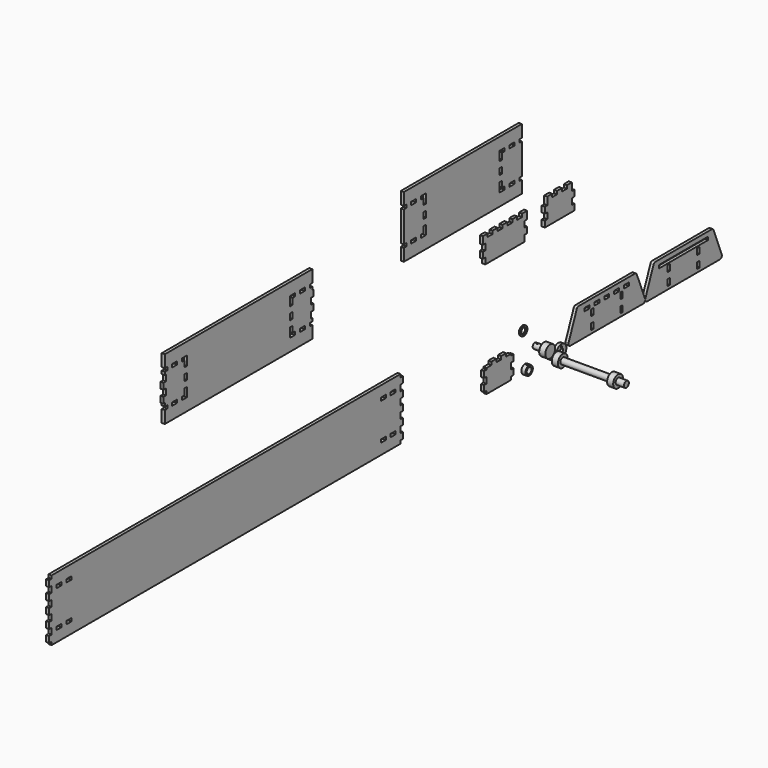
from build123d import *

# Parameters (mm, degrees)
F0_W      = 152.4
F0_H      = 101.6
F0_W_2    = 6.35
F0_H_2    = 12.7
F1_DEPTH  = 6.35
F2_W      = 152.4
F2_H      = 101.6
F2_W_2    = 6.35
F2_H_2    = 12.7
F2_W_3    = 127
F2_H_3    = 6.35
F3_DEPTH  = 6.35
F5_DEPTH  = 6.35
F6_W      = 12.7
F6_H      = 6.35
F7_DEPTH  = 6.35
F8_R      = 5.715
F9_DEPTH  = 19.05
F10_R     = 5.715
F11_DEPTH = 17.145
F12_R     = 12.7
F12_R_2   = 5.715
F13_DEPTH = 12.7
F14_R     = 6.35
F15_DEPTH = 101.6
F16_R     = 12.7
F16_R_2   = 6.35
F17_DEPTH = 12.7
F18_R     = 6.35
F19_DEPTH = 17.145
F20_R     = 12.7
F20_R_2   = 5.715
F21_DEPTH = 12.7
F22_R     = 1.5875
F23_DEPTH = 127.001
F24_R     = 9.525
F25_DEPTH = 8.4666666667
F26_R     = 1.5875
F27_DEPTH = 127.001
F28_R     = 6.35
F29_DEPTH = 8.4676667667
F30_R     = 9.525
F30_R_2   = 6.35
F31_DEPTH = 2.38125
F35_DEPTH = 6.35
F37_DEPTH = 6.35
F38_W     = 12.7
F38_H     = 6.35
F38_W_2   = 6.35
F38_H_2   = 12.7
F39_DEPTH = 6.35
F40_W     = 3.175
F40_H     = 12.7
F40_H_2   = 6.35
F41_DEPTH = 6.35
F42_W     = 152.4
F42_H     = 38.1
F43_DEPTH = 6.35
F44_W     = 152.4
F44_H     = 38.1
F45_DEPTH = 6.35
F47_DEPTH = 6.35
F48_R     = 5.08
F50_DEPTH = 6.35
F51_R     = 5.08
F52_R     = 12.7
F52_R_2   = 1.524
F52_R_3   = 4.445
F53_DEPTH = 6.35


# Not quite as in the source:
# - a feature names something its author has since deleted; it is built from what else it names


with BuildPart() as f1:
    # F0 (on Right) → F1 (new body)
    with BuildSketch(Plane.YZ):
        with Locations((76.2, 50.8)):
            Rectangle(F0_W, F0_H)
        with Locations((38.1, 12.7)):
            Rectangle(F0_W_2, F0_H_2, mode=Mode.SUBTRACT)
        with Locations((38.1, 38.1)):
            Rectangle(F0_W_2, F0_H_2, mode=Mode.SUBTRACT)
        Polygon((19.05, 53.975), (25.4, 53.975), (31.75, 53.975), (31.75, 50.8), (31.75, 47.625), (25.4, 47.625), (19.05, 47.625), (19.05, 50.8), align=None, mode=Mode.SUBTRACT)
        Polygon((44.45, 53.975), (50.8, 53.975), (57.15, 53.975), (57.15, 50.8), (57.15, 47.625), (50.8, 47.625), (44.45, 47.625), (44.45, 50.8), align=None, mode=Mode.SUBTRACT)
        Polygon((69.85, 53.975), (76.2, 53.975), (82.55, 53.975), (82.55, 50.8), (82.55, 47.625), (76.2, 47.625), (69.85, 47.625), (69.85, 50.8), align=None, mode=Mode.SUBTRACT)
        with Locations((114.3, 12.7)):
            Rectangle(F0_W_2, F0_H_2, mode=Mode.SUBTRACT)
        Polygon((95.25, 53.975), (101.6, 53.975), (107.95, 53.975), (107.95, 50.8), (107.95, 47.625), (101.6, 47.625), (95.25, 47.625), (95.25, 50.8), align=None, mode=Mode.SUBTRACT)
        with Locations((114.3, 38.1)):
            Rectangle(F0_W_2, F0_H_2, mode=Mode.SUBTRACT)
        Polygon((120.65, 53.975), (127, 53.975), (133.35, 53.975), (133.35, 50.8), (133.35, 47.625), (127, 47.625), (120.65, 47.625), (120.65, 50.8), align=None, mode=Mode.SUBTRACT)
    extrude(amount=F1_DEPTH)

    # F44 (on face) → F45 (cut, through all)
    with BuildSketch(Plane(origin=(0, 0, 0), x_dir=(0, -1, 0), z_dir=(-1, 0, 0))):
        with Locations((-76.2, 82.55)):
            Rectangle(F44_W, F44_H)
    extrude(amount=-F45_DEPTH, mode=Mode.SUBTRACT)

    # F49 (on face) → F50 (join)
    with BuildSketch(Plane(origin=(0, 0, 0), x_dir=(0, -1, 0), z_dir=(-1, 0, 0))):
        Polygon((-152.4, 0), (-152.4, 63.5), (-177.8, 0), align=None)
        Polygon((25.4, 0), (0, 63.5), (0, 0), align=None)
    extrude(amount=-F50_DEPTH)

    # F51
    f51_edges = [f1.edges().sort_by_distance(p)[0] for p in [
        (3.175, 152.4, 63.5),
        (3.175, 0, 63.5),
        (3.175, -25.4, 0),
        (3.175, 177.8, 0),
    ]]
    fillet(f51_edges, radius=F51_R)


with BuildPart() as f3:
    # F2 (on Right) → F3 (new body)
    with BuildSketch(Plane.YZ):
        with Locations((274.5815088749, 50.8)):
            Rectangle(F2_W, F2_H)
        with Locations((236.4815088749, 12.7)):
            Rectangle(F2_W_2, F2_H_2, mode=Mode.SUBTRACT)
        with Locations((236.4815088749, 38.1)):
            Rectangle(F2_W_2, F2_H_2, mode=Mode.SUBTRACT)
        with Locations((274.5815088749, 50.8)):
            Rectangle(F2_W_3, F2_H_3, mode=Mode.SUBTRACT)
        with Locations((312.6815088749, 12.7)):
            Rectangle(F2_W_2, F2_H_2, mode=Mode.SUBTRACT)
        with Locations((312.6815088749, 38.1)):
            Rectangle(F2_W_2, F2_H_2, mode=Mode.SUBTRACT)
    extrude(amount=F3_DEPTH)

    # F42 (on face) → F43 (cut, through all)
    with BuildSketch(Plane(origin=(0, 0, 0), x_dir=(0, -1, 0), z_dir=(-1, 0, 0))):
        with Locations((-274.5815088749, 82.55)):
            Rectangle(F42_W, F42_H)
    extrude(amount=-F43_DEPTH, mode=Mode.SUBTRACT)

    # F46 (on face) → F47 (join)
    with BuildSketch(Plane(origin=(0, 0, 0), x_dir=(0, -1, 0), z_dir=(-1, 0, 0))):
        Polygon((-350.7815088749, 0), (-350.7815088749, 63.5), (-376.1815088749, 0), align=None)
        Polygon((-172.9815088749, 0), (-198.3815088749, 63.5), (-198.3815088749, 0), align=None)
    extrude(amount=-F47_DEPTH)

    # F48
    f48_edges = [f3.edges().sort_by_distance(p)[0] for p in [
        (3.175, 350.781509, 63.5),
        (3.175, 198.381509, 63.5),
        (3.175, 376.181509, 0),
        (3.175, 172.981509, 0),
    ]]
    fillet(f48_edges, radius=F48_R)


with BuildPart() as f5:
    # F4 (on Right) → F5 (new body)
    with BuildSketch(Plane.YZ):
        Polygon((-234.6794404593, 0), (-171.1794404593, 0), (-171.1794404593, 6.35), (-164.8294404593, 6.35), (-164.8294404593, 19.05), (-171.1794404593, 19.05), (-171.1794404593, 31.75), (-164.8294404593, 31.75), (-164.8294404593, 44.45), (-171.1794404593, 44.45), (-171.1794404593, 47.625), (-183.8794404593, 47.625), (-183.8794404593, 53.975), (-196.5794404593, 53.975), (-196.5794404593, 47.625), (-202.9294404593, 47.625), (-209.2794404593, 47.625), (-209.2794404593, 53.975), (-221.9794404593, 53.975), (-221.9794404593, 47.625), (-234.6794404593, 47.625), (-234.6794404593, 44.45), (-241.0294404593, 44.45), (-241.0294404593, 31.75), (-234.6794404593, 31.75), (-234.6794404593, 19.05), (-241.0294404593, 19.05), (-241.0294404593, 6.35), (-234.6794404593, 6.35), align=None)
    extrude(amount=F5_DEPTH)


with BuildPart() as f7:
    # F6 (on Right) → F7 (new body)
    with BuildSketch(Plane.YZ):
        Polygon((-1358.3947817802, 0), (-456.6947817802, 0), (-456.6947817802, 6.35), (-450.3447817802, 6.35), (-450.3447817802, 19.05), (-456.6947817802, 19.05), (-456.6947817802, 22.225), (-456.6947817802, 28.575), (-456.6947817802, 31.75), (-450.3447817802, 31.75), (-450.3447817802, 44.45), (-456.6947817802, 44.45), (-456.6947817802, 57.15), (-450.3447817802, 57.15), (-450.3447817802, 69.85), (-456.6947817802, 69.85), (-456.6947817802, 82.55), (-450.3447817802, 82.55), (-450.3447817802, 95.25), (-456.6947817802, 95.25), (-456.6947817802, 98.425), (-456.6947817802, 104.775), (-456.6947817802, 107.95), (-450.3447817802, 107.95), (-450.3447817802, 120.65), (-456.6947817802, 120.65), (-456.6947817802, 127), (-1358.3947817802, 127), (-1358.3947817802, 120.65), (-1364.7447817802, 120.65), (-1364.7447817802, 107.95), (-1358.3947817802, 107.95), (-1358.3947817802, 104.775), (-1358.3947817802, 98.425), (-1358.3947817802, 95.25), (-1364.7447817802, 95.25), (-1364.7447817802, 82.55), (-1358.3947817802, 82.55), (-1358.3947817802, 69.85), (-1364.7447817802, 69.85), (-1364.7447817802, 57.15), (-1358.3947817802, 57.15), (-1358.3947817802, 44.45), (-1364.7447817802, 44.45), (-1364.7447817802, 31.75), (-1358.3947817802, 31.75), (-1358.3947817802, 28.575), (-1358.3947817802, 22.225), (-1358.3947817802, 19.05), (-1364.7447817802, 19.05), (-1364.7447817802, 6.35), (-1358.3947817802, 6.35), align=None)
        with Locations((-1339.3447817802, 25.4)):
            Rectangle(F6_W, F6_H, mode=Mode.SUBTRACT)
        with Locations((-1313.9447817802, 25.4)):
            Rectangle(F6_W, F6_H, mode=Mode.SUBTRACT)
        with Locations((-501.1447817802, 25.4)):
            Rectangle(F6_W, F6_H, mode=Mode.SUBTRACT)
        with Locations((-475.7447817802, 25.4)):
            Rectangle(F6_W, F6_H, mode=Mode.SUBTRACT)
        with Locations((-1339.3447817802, 101.6)):
            Rectangle(F6_W, F6_H, mode=Mode.SUBTRACT)
        with Locations((-1313.9447817802, 101.6)):
            Rectangle(F6_W, F6_H, mode=Mode.SUBTRACT)
        with Locations((-501.1447817802, 101.6)):
            Rectangle(F6_W, F6_H, mode=Mode.SUBTRACT)
        with Locations((-475.7447817802, 101.6)):
            Rectangle(F6_W, F6_H, mode=Mode.SUBTRACT)
    extrude(amount=F7_DEPTH)


with BuildPart() as f9:
    # F8 (on Right) → F9 (new body)
    with BuildSketch(Plane.YZ):
        with Locations((-101.6, 32.0885106921)):
            Circle(F8_R)
    extrude(amount=F9_DEPTH)

    # F20 (on face) → F21 (join)
    with BuildSketch(Plane.YZ.offset(19.05)):
        with Locations((-101.6, 32.0885106921)):
            Circle(F20_R)
        with Locations((-101.6, 32.0885106921)):
            Circle(F20_R_2, mode=Mode.SUBTRACT)
        with Locations((-101.6, 32.0885106921)):
            Circle(F20_R_2)
    extrude(amount=F21_DEPTH)

    # F22 (on Top) → F23 (cut, through all)
    with BuildSketch(Plane.XY):
        with Locations((4.7625, -101.6)):
            Circle(F22_R)
    extrude(amount=F23_DEPTH, mode=Mode.SUBTRACT)


with BuildPart() as f11:
    # F10 (on Right) → F11 (new body)
    with BuildSketch(Plane.YZ):
        with Locations((-66.7278746938, 0)):
            Circle(F10_R)
    extrude(amount=F11_DEPTH)

    # F12 (on face) → F13 (join)
    with BuildSketch(Plane.YZ.offset(17.145)):
        with Locations((-66.7278746938, 0)):
            Circle(F12_R)
        with Locations((-66.7278746938, 0)):
            Circle(F12_R_2, mode=Mode.SUBTRACT)
        with Locations((-66.7278746938, 0)):
            Circle(F12_R_2)
    extrude(amount=F13_DEPTH)

    # F14 (on face) → F15 (join)
    with BuildSketch(Plane.YZ.offset(29.845)):
        with Locations((-66.7278746938, 0)):
            Circle(F14_R)
    extrude(amount=F15_DEPTH)

    # F16 (on face) → F17 (join)
    with BuildSketch(Plane.YZ.offset(131.445)):
        with Locations((-66.7278746938, 0)):
            Circle(F16_R)
        with Locations((-66.7278746938, 0)):
            Circle(F16_R_2, mode=Mode.SUBTRACT)
        with Locations((-66.7278746938, 0)):
            Circle(F16_R_2)
    extrude(amount=F17_DEPTH)

    # F18 (on face) → F19 (join)
    with BuildSketch(Plane.YZ.offset(144.145)):
        with Locations((-66.7278746938, 0)):
            Circle(F18_R)
    extrude(amount=F19_DEPTH)


with BuildPart() as f25:
    # F24 (on Right) → F25 (new body)
    with BuildSketch(Plane.YZ):
        with Locations((-127, 0)):
            Circle(F24_R)
    extrude(amount=F25_DEPTH)

    # F26 (on Top) → F27 (cut, through all)
    with BuildSketch(Plane.XY):
        with Locations((4.2333333333, -127)):
            Circle(F26_R)
    extrude(amount=F27_DEPTH, mode=Mode.SUBTRACT)

    # F28 (on face) → F29 (cut, through all)
    with BuildSketch(Plane(origin=(0, 0, 0), x_dir=(0, -1, 0), z_dir=(-1, 0, 0))):
        with Locations((127, 0)):
            Circle(F28_R)
    extrude(amount=-F29_DEPTH, mode=Mode.SUBTRACT)


with BuildPart() as f31:
    # F30 (on Right) → F31 (new body)
    with BuildSketch(Plane.YZ):
        with Locations((-133.449241519, 72.6503282785)):
            Circle(F30_R)
        with Locations((-133.449241519, 72.6503282785)):
            Circle(F30_R_2, mode=Mode.SUBTRACT)
    extrude(amount=F31_DEPTH)


with BuildPart() as f32_1:
    # F32: copy of F5
    add(f5.part)


with BuildPart() as f35:
    # F34 (on Right) → F35 (new body)
    with BuildSketch(Plane.YZ):
        Polygon((-237.713524918, 249.9757648349), (-237.713524918, 237.2757648349), (-136.113524918, 237.2757648349), (-136.113524918, 249.9757648349), (-129.763524918, 249.9757648349), (-129.763524918, 262.6757648349), (-136.113524918, 262.6757648349), (-136.113524918, 275.3757648349), (-129.763524918, 275.3757648349), (-129.763524918, 291.2507648349), (-142.463524918, 291.2507648349), (-142.463524918, 284.9007648349), (-155.163524918, 284.9007648349), (-155.163524918, 291.2507648349), (-167.863524918, 291.2507648349), (-167.863524918, 284.9007648349), (-180.563524918, 284.9007648349), (-180.563524918, 291.2507648349), (-193.263524918, 291.2507648349), (-193.263524918, 284.9007648349), (-205.963524918, 284.9007648349), (-205.963524918, 291.2507648349), (-218.663524918, 291.2507648349), (-218.663524918, 284.9007648349), (-231.363524918, 284.9007648349), (-231.363524918, 291.2507648349), (-244.063524918, 291.2507648349), (-244.063524918, 275.3757648349), (-237.713524918, 275.3757648349), (-237.713524918, 262.6757648349), (-244.063524918, 262.6757648349), (-244.063524918, 249.9757648349), align=None)
    extrude(amount=F35_DEPTH)


with BuildPart() as f37:
    # F36 (on Right) → F37 (new body)
    with BuildSketch(Plane.YZ):
        Polygon((-83.9351456323, 254.5199484468), (-83.9351456323, 241.8199484468), (-7.7351456323, 241.8199484468), (-7.7351456323, 254.5199484468), (-14.0851456323, 254.5199484468), (-14.0851456323, 267.2199484468), (-7.7351456323, 267.2199484468), (-7.7351456323, 279.9199484468), (-14.0851456323, 279.9199484468), (-14.0851456323, 295.7949484468), (-26.7851456323, 295.7949484468), (-26.7851456323, 289.4449484468), (-39.4851456323, 289.4449484468), (-39.4851456323, 295.7949484468), (-52.1851456323, 295.7949484468), (-52.1851456323, 289.4449484468), (-64.8851456323, 289.4449484468), (-64.8851456323, 295.7949484468), (-77.5851456323, 295.7949484468), (-77.5851456323, 279.9199484468), (-83.9351456323, 279.9199484468), (-83.9351456323, 267.2199484468), (-77.5851456323, 267.2199484468), (-77.5851456323, 254.5199484468), align=None)
    extrude(amount=F37_DEPTH)


with BuildPart() as f39:
    # F38 (on Right) → F39 (new body)
    with BuildSketch(Plane.YZ):
        Polygon((-441.788833046, 353.0291121978), (-448.138833046, 353.0291121978), (-448.138833046, 327.6291121978), (-143.338833046, 327.6291121978), (-143.338833046, 353.0291121978), (-149.688833046, 353.0291121978), (-149.688833046, 359.3791121978), (-143.338833046, 359.3791121978), (-143.338833046, 422.8791121978), (-149.688833046, 422.8791121978), (-149.688833046, 429.2291121978), (-143.338833046, 429.2291121978), (-143.338833046, 454.6291121978), (-448.138833046, 454.6291121978), (-448.138833046, 429.2291121978), (-441.788833046, 429.2291121978), (-429.088833046, 429.2291121978), (-416.388833046, 429.2291121978), (-403.688833046, 429.2291121978), (-390.988833046, 429.2291121978), (-390.988833046, 422.8791121978), (-390.988833046, 410.1791121978), (-390.988833046, 397.4791121978), (-390.988833046, 384.7791121978), (-390.988833046, 372.0791121978), (-390.988833046, 359.3791121978), (-390.988833046, 353.0291121978), (-403.688833046, 353.0291121978), (-416.388833046, 353.0291121978), (-429.088833046, 353.0291121978), align=None)
        with Locations((-168.738833046, 356.2041121978)):
            Rectangle(F38_W, F38_H, mode=Mode.SUBTRACT)
        Polygon((-187.788833046, 359.3791121978), (-187.788833046, 353.0291121978), (-200.488833046, 353.0291121978), (-200.488833046, 359.3791121978), (-200.488833046, 372.0791121978), (-194.138833046, 372.0791121978), (-194.138833046, 359.3791121978), align=None, mode=Mode.SUBTRACT)
        with Locations((-197.313833046, 391.1291121978)):
            Rectangle(F38_W_2, F38_H_2, mode=Mode.SUBTRACT)
        Polygon((-194.138833046, 410.1791121978), (-200.488833046, 410.1791121978), (-200.488833046, 422.8791121978), (-200.488833046, 429.2291121978), (-187.788833046, 429.2291121978), (-187.788833046, 422.8791121978), (-194.138833046, 422.8791121978), align=None, mode=Mode.SUBTRACT)
        with Locations((-168.738833046, 426.0541121978)):
            Rectangle(F38_W, F38_H, mode=Mode.SUBTRACT)
        Polygon((-441.788833046, 359.3791121978), (-441.788833046, 353.0291121978), (-429.088833046, 353.0291121978), (-429.088833046, 359.3791121978), (-416.388833046, 359.3791121978), (-416.388833046, 353.0291121978), (-403.688833046, 353.0291121978), (-403.688833046, 359.3791121978), (-397.338833046, 359.3791121978), (-397.338833046, 372.0791121978), (-390.988833046, 372.0791121978), (-390.988833046, 384.7791121978), (-397.338833046, 384.7791121978), (-397.338833046, 397.4791121978), (-390.988833046, 397.4791121978), (-390.988833046, 410.1791121978), (-397.338833046, 410.1791121978), (-397.338833046, 422.8791121978), (-403.688833046, 422.8791121978), (-403.688833046, 429.2291121978), (-416.388833046, 429.2291121978), (-416.388833046, 422.8791121978), (-429.088833046, 422.8791121978), (-429.088833046, 429.2291121978), (-441.788833046, 429.2291121978), (-441.788833046, 422.8791121978), (-448.138833046, 422.8791121978), (-448.138833046, 359.3791121978), align=None)
    extrude(amount=F39_DEPTH)


with BuildPart() as f41:
    # F40 (on Right) → F41 (new body)
    with BuildSketch(Plane.YZ):
        Polygon((-1062.6830654318, 321.5943043449), (-1062.6830654318, 315.2443043449), (-1059.5080654318, 315.2443043449), (-1059.5080654318, 308.8943043449), (-1046.8080654318, 308.8943043449), (-1046.8080654318, 315.2443043449), (-1034.1080654318, 315.2443043449), (-1034.1080654318, 308.8943043449), (-1021.4080654318, 308.8943043449), (-1021.4080654318, 315.2443043449), (-1015.0580654318, 315.2443043449), (-1015.0580654318, 327.9443043449), (-1008.7080654318, 327.9443043449), (-1008.7080654318, 340.6443043449), (-1015.0580654318, 340.6443043449), (-1015.0580654318, 353.3443043449), (-1008.7080654318, 353.3443043449), (-1008.7080654318, 366.0443043449), (-1015.0580654318, 366.0443043449), (-1015.0580654318, 378.7443043449), (-1021.4080654318, 378.7443043449), (-1021.4080654318, 385.0943043449), (-1034.1080654318, 385.0943043449), (-1034.1080654318, 378.7443043449), (-1046.8080654318, 378.7443043449), (-1046.8080654318, 385.0943043449), (-1059.5080654318, 385.0943043449), (-1059.5080654318, 378.7443043449), (-1062.6830654318, 378.7443043449), (-1062.6830654318, 372.3943043449), (-1062.6830654318, 359.6943043449), (-1062.6830654318, 346.9943043449), (-1062.6830654318, 334.2943043449), align=None)
        with Locations((-1064.2705654318, 353.3443043449)):
            Rectangle(F40_W, F40_H)
        with Locations((-1067.4455654318, 353.3443043449)):
            Rectangle(F40_W, F40_H)
        with Locations((-1064.2705654318, 327.9443043449)):
            Rectangle(F40_W, F40_H)
        with Locations((-1067.4455654318, 327.9443043449)):
            Rectangle(F40_W, F40_H)
        with Locations((-1064.2705654318, 318.4193043449)):
            Rectangle(F40_W, F40_H_2)
        with Locations((-1064.2705654318, 375.5693043449)):
            Rectangle(F40_W, F40_H_2)
        Polygon((-1065.8580654318, 283.4943043449), (-684.8580654318, 283.4943043449), (-684.8580654318, 308.8943043449), (-688.0330654318, 308.8943043449), (-691.2080654318, 308.8943043449), (-703.9080654318, 308.8943043449), (-716.6080654318, 308.8943043449), (-729.3080654318, 308.8943043449), (-735.6580654318, 308.8943043449), (-742.0080654318, 308.8943043449), (-742.0080654318, 315.2443043449), (-742.0080654318, 327.9443043449), (-742.0080654318, 340.6443043449), (-742.0080654318, 353.3443043449), (-742.0080654318, 366.0443043449), (-742.0080654318, 378.7443043449), (-742.0080654318, 385.0943043449), (-735.6580654318, 385.0943043449), (-729.3080654318, 385.0943043449), (-716.6080654318, 385.0943043449), (-703.9080654318, 385.0943043449), (-691.2080654318, 385.0943043449), (-688.0330654318, 385.0943043449), (-684.8580654318, 385.0943043449), (-684.8580654318, 391.4443043449), (-684.8580654318, 404.1443043449), (-684.8580654318, 410.4943043449), (-691.2080654318, 410.4943043449), (-1065.8580654318, 410.4943043449), (-1065.8580654318, 385.0943043449), (-1062.6830654318, 385.0943043449), (-1059.5080654318, 385.0943043449), (-1046.8080654318, 385.0943043449), (-1034.1080654318, 385.0943043449), (-1021.4080654318, 385.0943043449), (-1015.0580654318, 385.0943043449), (-1008.7080654318, 385.0943043449), (-1008.7080654318, 378.7443043449), (-1008.7080654318, 366.0443043449), (-1008.7080654318, 353.3443043449), (-1008.7080654318, 340.6443043449), (-1008.7080654318, 327.9443043449), (-1008.7080654318, 315.2443043449), (-1008.7080654318, 308.8943043449), (-1015.0580654318, 308.8943043449), (-1021.4080654318, 308.8943043449), (-1034.1080654318, 308.8943043449), (-1046.8080654318, 308.8943043449), (-1059.5080654318, 308.8943043449), (-1062.6830654318, 308.8943043449), (-1065.8580654318, 308.8943043449), align=None)
        Polygon((-691.2080654318, 315.2443043449), (-688.0330654318, 315.2443043449), (-688.0330654318, 321.5943043449), (-688.0330654318, 334.2943043449), (-688.0330654318, 346.9943043449), (-688.0330654318, 359.6943043449), (-688.0330654318, 372.3943043449), (-688.0330654318, 378.7443043449), (-691.2080654318, 378.7443043449), (-691.2080654318, 385.0943043449), (-703.9080654318, 385.0943043449), (-703.9080654318, 378.7443043449), (-716.6080654318, 378.7443043449), (-716.6080654318, 385.0943043449), (-729.3080654318, 385.0943043449), (-729.3080654318, 378.7443043449), (-735.6580654318, 378.7443043449), (-735.6580654318, 366.0443043449), (-742.0080654318, 366.0443043449), (-742.0080654318, 353.3443043449), (-735.6580654318, 353.3443043449), (-735.6580654318, 340.6443043449), (-742.0080654318, 340.6443043449), (-742.0080654318, 327.9443043449), (-735.6580654318, 327.9443043449), (-735.6580654318, 315.2443043449), (-729.3080654318, 315.2443043449), (-729.3080654318, 308.8943043449), (-716.6080654318, 308.8943043449), (-716.6080654318, 315.2443043449), (-703.9080654318, 315.2443043449), (-703.9080654318, 308.8943043449), (-691.2080654318, 308.8943043449), align=None)
        with Locations((-686.4455654318, 375.5693043449)):
            Rectangle(F40_W, F40_H_2)
        with Locations((-686.4455654318, 366.0443043449)):
            Rectangle(F40_W, F40_H)
        with Locations((-683.2705654318, 366.0443043449)):
            Rectangle(F40_W, F40_H)
        with Locations((-686.4455654318, 340.6443043449)):
            Rectangle(F40_W, F40_H)
        with Locations((-683.2705654318, 340.6443043449)):
            Rectangle(F40_W, F40_H)
        with Locations((-686.4455654318, 318.4193043449)):
            Rectangle(F40_W, F40_H_2)
    extrude(amount=F41_DEPTH)


with BuildPart() as f53:
    # F52 (on Right) → F53 (new body)
    with BuildSketch(Plane.YZ):
        with Locations((-40.9202546468, 0)):
            Circle(F52_R)
        with Locations((-40.9202546468, -7.3025)):
            Circle(F52_R_2, mode=Mode.SUBTRACT)
        with Locations((-40.9202546468, 0)):
            Circle(F52_R_3, mode=Mode.SUBTRACT)
        with Locations((-40.9202546468, 7.3025)):
            Circle(F52_R_2, mode=Mode.SUBTRACT)
    extrude(amount=F53_DEPTH)


solid = Compound([f1.part, f3.part, f5.part, f7.part, f9.part, f11.part, f25.part, f31.part, f35.part, f37.part, f39.part, f41.part, f53.part])
